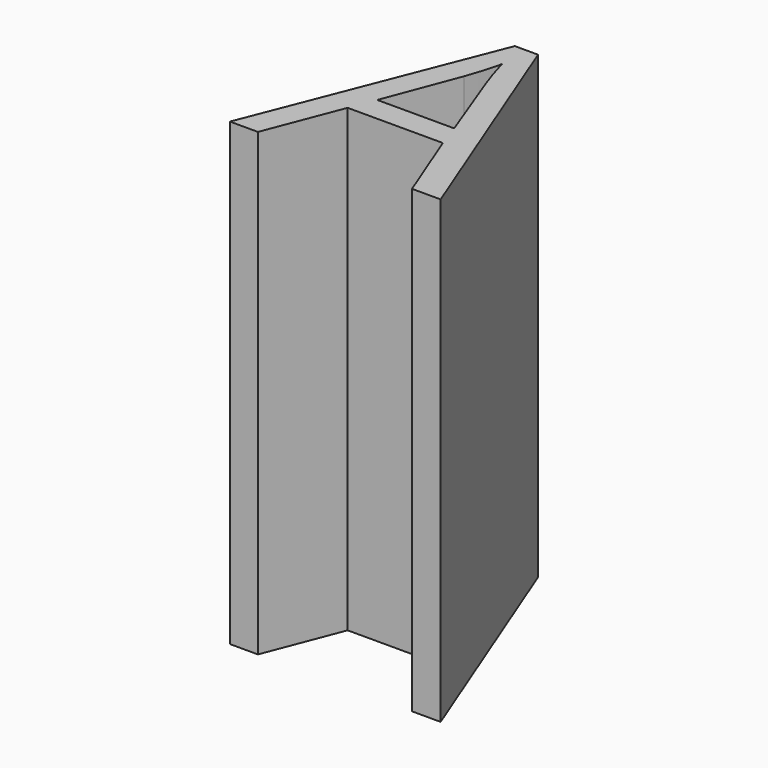
from build123d import *

# Parameters (mm, degrees)
F0_TEXT_SIZE = 91.9108718841
F1_DEPTH     = 127


# Not quite as in the source:
# - Text() gives the source's letters only with a copy of the font that has no kerning and outlines rounded to 1/6400 em; it was checked with that copy


with BuildPart() as f1:
    # F0 (on Top) → F1 (new body)
    with BuildSketch(Plane.XY):
        with Locations((-27.3831021041, -22.9618716985)):
            Text('A', F0_TEXT_SIZE, font='Open Sans', text_align=(TextAlign.LEFT, TextAlign.BOTTOM))
    extrude(amount=F1_DEPTH)


solid = f1.part
